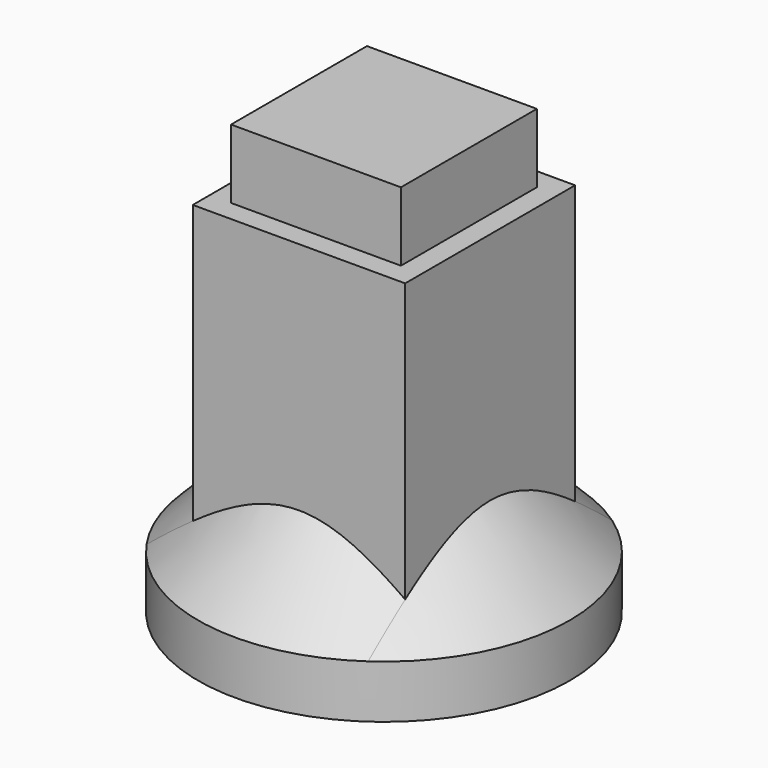
from build123d import *

# Parameters (mm, degrees)
F0_W     = 120
F0_H     = 120
F1_DEPTH = 246.38
F2_W     = 120
F2_H     = 120
F2_W_2   = 96
F2_H_2   = 96
F3_DEPTH = 39
F4_R     = 105
F4_W     = 120
F4_H     = 120
F5_DEPTH = 100
F7_DEPTH = 80


# Not quite as in the source:
# - a fillet or chamfer that OpenCascade refuses, or shapes differently, is made with other operations: its cross-section is extruded or revolved along the edge and cut away or added


with BuildPart() as f1:
    # F0 (on Top) → F1 (new body)
    with BuildSketch(Plane.XY):
        with Locations((60, 60)):
            Rectangle(F0_W, F0_H)
    extrude(amount=F1_DEPTH)

    # F2 (on face) → F3 (cut)
    with BuildSketch(Plane.XY.offset(246.38)):
        with Locations((60, 60)):
            Rectangle(F2_W, F2_H)
        with Locations((60, 60)):
            Rectangle(F2_W_2, F2_H_2, mode=Mode.SUBTRACT)
    extrude(amount=-F3_DEPTH, mode=Mode.SUBTRACT)

    # F4 (on face) → F5 (join)
    with BuildSketch(Plane(origin=(0, 0, 0), x_dir=(1, 0, 0), z_dir=(0, 0, -1))):
        with Locations((60, -60)):
            Circle(F4_R)
        with Locations((60, -60)):
            Rectangle(F4_W, F4_H, mode=Mode.SUBTRACT)
    extrude(amount=-F5_DEPTH)

    # F6: chamfer of 70 on 1 edges, made by hand


with BuildPart() as f6_tool2:
    # F6_s3 → F6_t4 (revolve)
    with BuildSketch(Plane.XZ.offset(-60)):
        Polygon((95, 100), (165, 30), (165, 100), align=None)
    revolve(axis=Axis((60, 60, 100), (0, 0, -1)))

    split(bisect_by=Plane.YZ.offset(120), keep=Keep.TOP)


with BuildPart() as f1_1:
    add(f1.part)

    # F6_t1: cut F6_tool2
    add(f6_tool2.part, mode=Mode.SUBTRACT)


with BuildPart() as f6_tool7:
    # F6_s8 → F6_t9 (revolve)
    with BuildSketch(Plane.XZ.offset(-60)):
        Polygon((95, 100), (165, 30), (165, 100), align=None)
    revolve(axis=Axis((60, 60, 100), (0, 0, -1)))

    split(bisect_by=Plane.XZ, keep=Keep.TOP)


with BuildPart() as f1_2:
    add(f1_1.part)

    # F6_t6: cut F6_tool7
    add(f6_tool7.part, mode=Mode.SUBTRACT)


with BuildPart() as f6_tool12:
    # F6_s13 → F6_t14 (revolve)
    with BuildSketch(Plane.XZ.offset(-60)):
        Polygon((95, 100), (165, 30), (165, 100), align=None)
    revolve(axis=Axis((60, 60, 100), (0, 0, -1)))

    split(bisect_by=Plane.YZ, keep=Keep.BOTTOM)


with BuildPart() as f1_3:
    add(f1_2.part)

    # F6_t11: cut F6_tool12
    add(f6_tool12.part, mode=Mode.SUBTRACT)


with BuildPart() as f6_tool17:
    # F6_s18 → F6_t19 (revolve)
    with BuildSketch(Plane.XZ.offset(-60)):
        Polygon((95, 100), (165, 30), (165, 100), align=None)
    revolve(axis=Axis((60, 60, 100), (0, 0, -1)))

    split(bisect_by=Plane.XZ.offset(-120), keep=Keep.BOTTOM)


with BuildPart() as f1_4:
    add(f1_3.part)

    # F6_t16: cut F6_tool17
    add(f6_tool17.part, mode=Mode.SUBTRACT)


with BuildPart() as f7:
    # F7 (new): a face of the model
    f7_faces = [f1_4.part.faces().sort_by_distance(p)[0] for p in [
        (60, 118.3029437252, 207.38),
    ]]
    extrude(f7_faces, amount=F7_DEPTH)


solid = f1_4.part
